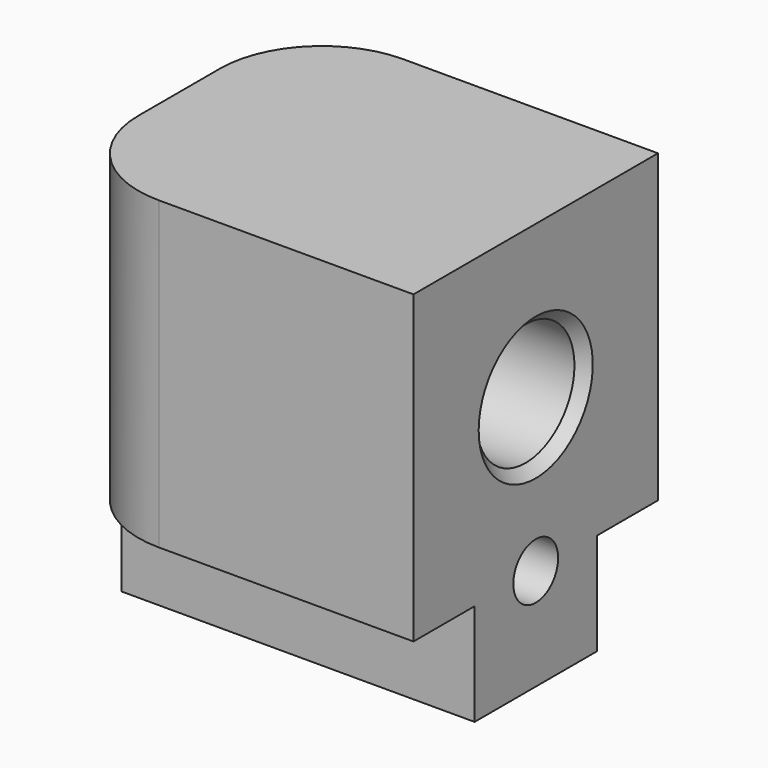
from build123d import *

# Parameters (mm, degrees)
F1_DEPTH       = 35
F3_D           = 12
F3_CSINK_D     = 14
F3_CSINK_ANGLE = 90
F4_T1_DEPTH    = 80
F5_D           = 5.5
F5_DEPTH       = 20
F5_TIP         = 1.6523667023


# Not quite as in the source:
# - a fillet or chamfer that OpenCascade refuses, or shapes differently, is made with other operations: its cross-section is extruded or revolved along the edge and cut away or added


with BuildPart() as f1:
    # F0 (on Right) → F1 (new body)
    with BuildSketch(Plane.YZ):
        Polygon((15, 30), (0, 30), (-15, 30), (-15, 0), (-7.5, 0), (-7.5, -10), (0, -10), (7.5, -10), (7.5, 0), (15, 0), align=None)
    extrude(amount=-F1_DEPTH)

    # F3 (through all)
    with Locations(Plane.YZ):
        with Locations((0, 15)):
            CounterSinkHole(F3_D / 2, F3_CSINK_D / 2, counter_sink_angle=F3_CSINK_ANGLE)

    # F4: fillet of radius 10 on 2 edges, made by hand

    # F4_s2 → F4_t1 (cut)
    with BuildSketch(Plane.XY.offset(-25)):
        with BuildLine():
            ThreePointArc((-25, 15), (-32.0710678119, 12.0710678119), (-35, 5))
            Line((-35, 5), (-35, 15))
            Line((-35, 15), (-25, 15))
        make_face()
        with BuildLine():
            ThreePointArc((-35, -5), (-32.0710678119, -12.0710678119), (-25, -15))
            Line((-25, -15), (-35, -15))
            Line((-35, -15), (-35, -5))
        make_face()
    extrude(amount=F4_T1_DEPTH, mode=Mode.SUBTRACT)

    # F5
    with Locations(Plane.YZ):
        with Locations((0, 0)):
            Hole(F5_D / 2, depth=F5_DEPTH)
            with Locations((0, 0, -(F5_DEPTH + F5_TIP / 2))):  # 118° drill point
                Cone(0, F5_D / 2, F5_TIP, mode=Mode.SUBTRACT)


solid = f1.part
